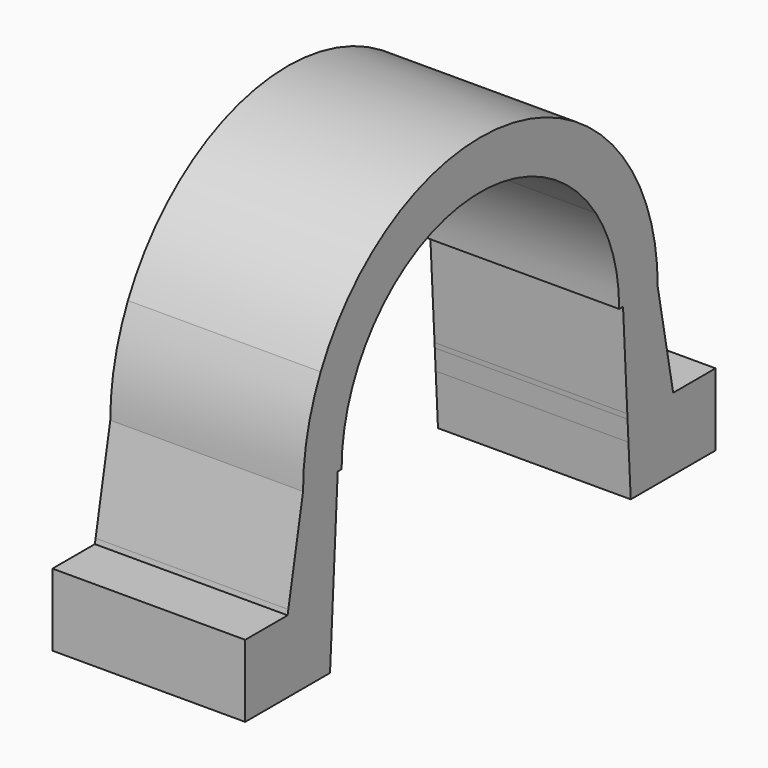
from build123d import *

# Parameters (mm, degrees)
F1_DEPTH = 20


with BuildPart() as f1:
    # F0 (on Right) → F1 (new body)
    with BuildSketch(Plane.YZ):
        with BuildLine():
            ThreePointArc((14.9666295471, 10), (17.2249721603, 5.2249721603), (18, 0))
            Line((18, 0), (18.5, 0))
            Line((18.5, 0), (23, 0))
            ThreePointArc((23, 0), (22.4207855469, 5.1291690811), (20.7123151772, 10))
            Line((20.7123151772, 10), (14.9666295471, 10))
        make_face()
        with BuildLine():
            ThreePointArc((-14.9666295471, 10), (0, 18), (14.9666295471, 10))
            Line((14.9666295471, 10), (20.7123151772, 10))
            ThreePointArc((20.7123151772, 10), (0, 23), (-20.7123151772, 10))
            Line((-20.7123151772, 10), (-14.9666295471, 10))
        make_face()
        with BuildLine():
            Line((23, 0), (18.5, 0))
            Line((18.5, 0), (19.0555555556, -10))
            Line((19.0555555556, -10), (20.7123151772, -10))
            ThreePointArc((20.7123151772, -10), (22.4207855469, -5.1291690811), (23, 0))
        make_face()
        with BuildLine():
            ThreePointArc((-18, 0), (-17.2249721603, 5.2249721603), (-14.9666295471, 10))
            Line((-14.9666295471, 10), (-20.7123151772, 10))
            ThreePointArc((-20.7123151772, 10), (-22.4207855469, 5.1291690811), (-23, 0))
            Line((-23, 0), (-18.5, 0))
            Line((-18.5, 0), (-18, 0))
        make_face()
        with BuildLine():
            Line((23, -10), (23, 0))
            ThreePointArc((23, 0), (22.4207855469, -5.1291690811), (20.7123151772, -10))
            Line((20.7123151772, -10), (23, -10))
        make_face()
        Polygon((24.9047619048, -10), (23, 0), (23, -10), align=None)
        with BuildLine():
            Line((20.7123151772, -10), (19.0555555556, -10))
            Line((19.0555555556, -10), (19.0833333333, -10.5))
            Line((19.0833333333, -10.5), (20.4633819297, -10.5))
            ThreePointArc((20.4633819297, -10.5), (20.5893663831, -10.2507556766), (20.7123151772, -10))
        make_face()
        with BuildLine():
            Line((-19.0555555556, -10), (-18.5, 0))
            Line((-18.5, 0), (-23, 0))
            ThreePointArc((-23, 0), (-22.4207855469, -5.1291690811), (-20.7123151772, -10))
            Line((-20.7123151772, -10), (-19.0555555556, -10))
        make_face()
        with BuildLine():
            Line((23, -10), (20.7123151772, -10))
            ThreePointArc((20.7123151772, -10), (20.5893663831, -10.2507556766), (20.4633819297, -10.5))
            Line((20.4633819297, -10.5), (23, -10.5))
            Line((23, -10.5), (23, -10))
        make_face()
        Polygon((24.9047619048, -10), (23, -10), (23, -10.5), (25, -10.5), align=None)
        with BuildLine():
            Line((20.4633819297, -10.5), (19.0833333333, -10.5))
            Line((19.0833333333, -10.5), (19.2032450764, -12.6584113749))
            ThreePointArc((19.2032450764, -12.6584113749), (19.862653635, -11.5963352217), (20.4633819297, -10.5))
        make_face()
        with BuildLine():
            ThreePointArc((-20.7123151772, -10), (-22.4207855469, -5.1291690811), (-23, 0))
            Line((-23, 0), (-24.9047619048, -10))
            Line((-24.9047619048, -10), (-20.7123151772, -10))
        make_face()
        with BuildLine():
            Line((-19.0833333333, -10.5), (-19.0555555556, -10))
            Line((-19.0555555556, -10), (-20.7123151772, -10))
            ThreePointArc((-20.7123151772, -10), (-20.5893663831, -10.2507556766), (-20.4633819297, -10.5))
            Line((-20.4633819297, -10.5), (-19.0833333333, -10.5))
        make_face()
        with BuildLine():
            Line((-19.5, -18), (-19.2032450764, -12.6584113749))
            ThreePointArc((-19.2032450764, -12.6584113749), (-19.862653635, -11.5963352217), (-20.4633819297, -10.5))
            Line((-20.4633819297, -10.5), (-25, -10.5))
            Line((-25, -10.5), (-30.5, -10.5))
            Line((-30.5, -10.5), (-30.5, -18))
            Line((-30.5, -18), (-19.5, -18))
        make_face()
        with BuildLine():
            ThreePointArc((-20.4633819297, -10.5), (-19.862653635, -11.5963352217), (-19.2032450764, -12.6584113749))
            Line((-19.2032450764, -12.6584113749), (-19.0833333333, -10.5))
            Line((-19.0833333333, -10.5), (-20.4633819297, -10.5))
        make_face()
        with BuildLine():
            Line((23, -10.5), (20.4633819297, -10.5))
            ThreePointArc((20.4633819297, -10.5), (19.862653635, -11.5963352217), (19.2032450764, -12.6584113749))
            Line((19.2032450764, -12.6584113749), (19.5, -18))
            Line((19.5, -18), (30.5, -18))
            Line((30.5, -18), (30.5, -10.5))
            Line((30.5, -10.5), (25, -10.5))
            Line((25, -10.5), (23, -10.5))
        make_face()
        with BuildLine():
            ThreePointArc((-20.4633819297, -10.5), (-20.5893663831, -10.2507556766), (-20.7123151772, -10))
            Line((-20.7123151772, -10), (-24.9047619048, -10))
            Line((-24.9047619048, -10), (-25, -10.5))
            Line((-25, -10.5), (-20.4633819297, -10.5))
        make_face()
    extrude(amount=F1_DEPTH)


solid = f1.part
